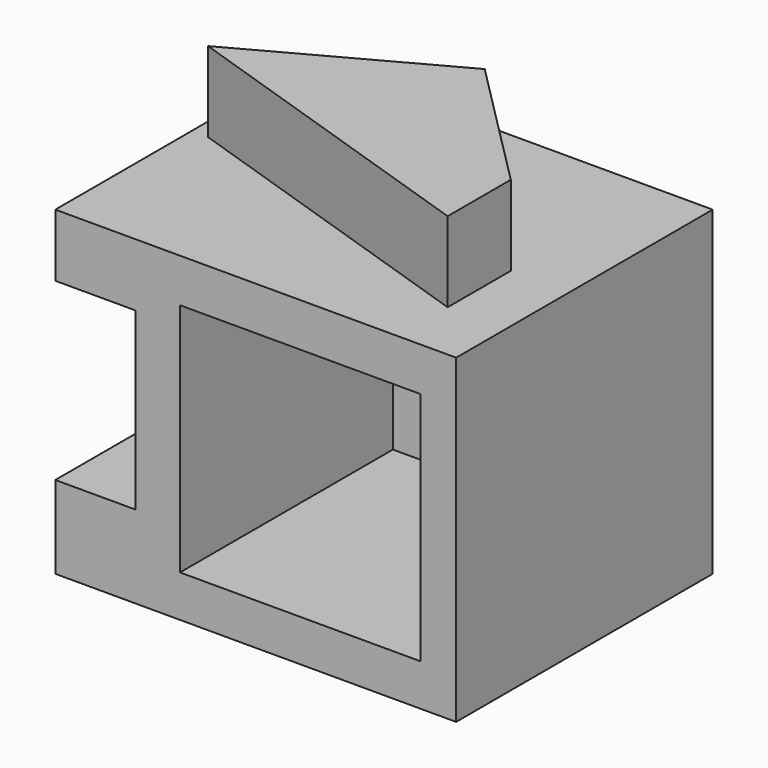
from build123d import *

# Parameters (mm, degrees)
F0_W     = 100
F0_H     = 100
F1_DEPTH = 100
F2_W     = 75.0674530864
F2_H     = 73.3678080142
F3_DEPTH = 83
F4_W     = 100
F4_H     = 25.7778791711
F5_DEPTH = 25
F6_W     = 100
F6_H     = 19.5503592491
F7_DEPTH = 25
F9_DEPTH = 25


# Not quite as in the source:
# - the program builds the solid bodies; features that only make, move or delete a surface that nothing else refers to are left out


with BuildPart() as f1:
    # F0 (on Front) → F1 (new body)
    with BuildSketch(Plane.XZ):
        with Locations((17.8484685719, 11.3331817091)):
            Rectangle(F0_W, F0_H)
    extrude(amount=F1_DEPTH)

    # F2 (on face) → F3 (cut)
    with BuildSketch(Plane.XZ.offset(100)):
        with Locations((19.2625932395, 11.0476631671)):
            Rectangle(F2_W, F2_H)
    extrude(amount=-F3_DEPTH, mode=Mode.SUBTRACT)

    # F4 (on face) → F5 (join)
    with BuildSketch(Plane(origin=(-32.1515314281, 0, 0), x_dir=(0, -1, 0), z_dir=(-1, 0, 0))):
        with Locations((50, -25.7778787054)):
            Rectangle(F4_W, F4_H)
    extrude(amount=F5_DEPTH)

    # F6 (on face) → F7 (join)
    with BuildSketch(Plane(origin=(-32.1515314281, 0, 0), x_dir=(0, -1, 0), z_dir=(-1, 0, 0))):
        with Locations((50, 51.5580020845)):
            Rectangle(F6_W, F6_H)
    extrude(amount=F7_DEPTH)

    # F8 (on face) → F9 (join)
    with BuildSketch(Plane.XY.offset(61.3331817091)):
        Polygon((8.1979809329, -14.2997056246), (-51.9804432988, -46.9225756824), (49.6200919151, -80.5339738727), (49.6200919151, -55.9161007404), align=None)
    extrude(amount=F9_DEPTH)


solid = f1.part
